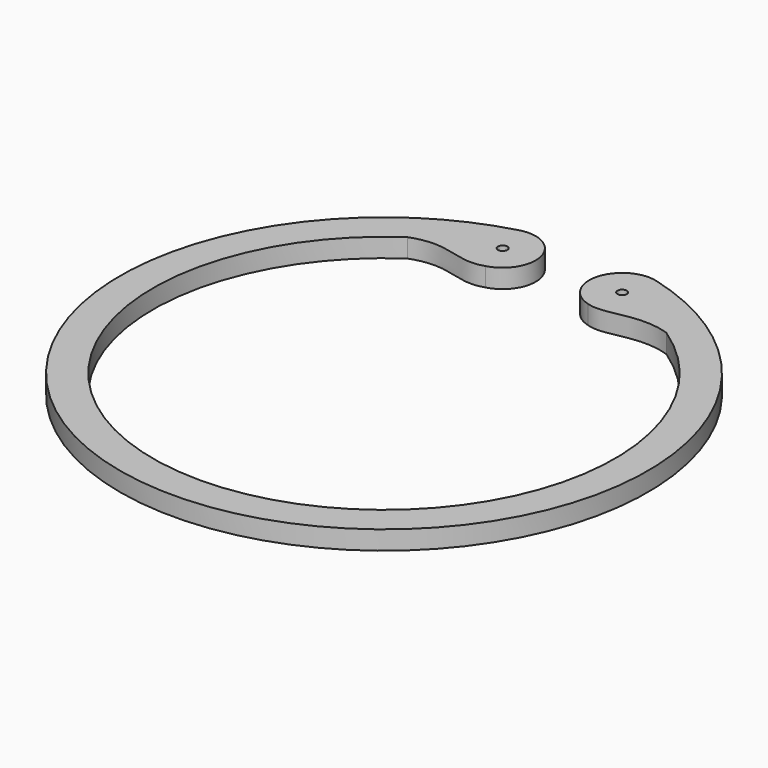
from build123d import *

# Parameters (mm, degrees)
F1_DEPTH = 1
F2_D     = 0.5
F2_DEPTH = 17
F2_TIP   = 0.1502151548


with BuildPart() as f1:
    # F0 (on Top) → F1 (new body)
    with BuildSketch(Plane.XY):
        with BuildLine():
            add(Edge.make_bspline(
                [(-6.8700691129, 10.142221176), (-8.399545307, 9.5712927005), (-10.6213726103, 7.7990288846), (-9.4482654422, 10.3310348046)],
                knots=[0.5589666429, 0.5589666429, 0.5589666429, 0.5589666429, 1, 1, 1, 1], degree=3))
            add(Edge.make_bspline(
                [(-2.7175999736, 10.142221176), (-4.1052754968, 9.659698233), (-4.9316076337, 10.8658171767), (-6.8700691129, 10.142221176)],
                knots=[0, 0, 0, 0, 0.5589666429, 0.5589666429, 0.5589666429, 0.5589666429], degree=3))
            Line((-2.7175999736, 10.142221176), (-3.6234666314, 13.522961568))
            ThreePointArc((-3.6234666314, 13.522961568), (-6.727900413, 12.2774327949), (-9.4482654422, 10.3310348046))
        make_face()
        with BuildLine():
            ThreePointArc((6.8700691129, 10.142221176), (0, -12.25), (-6.8700691129, 10.142221176))
            add(Edge.make_bspline(
                [(-6.8700691129, 10.142221176), (-8.399545307, 9.5712927005), (-10.6213726103, 7.7990288846), (-9.4482654422, 10.3310348046)],
                knots=[0.5589666429, 0.5589666429, 0.5589666429, 0.5589666429, 1, 1, 1, 1], degree=3))
            ThreePointArc((-9.4482654422, 10.3310348046), (0, -14), (9.4482654422, 10.3310348046))
            add(Edge.make_bspline(
                [(6.8700691129, 10.142221176), (8.3520722793, 9.6407168218), (10.2458875626, 8.1284232438), (9.4482654422, 10.3310348046)],
                knots=[0.5589666429, 0.5589666429, 0.5589666429, 0.5589666429, 1, 1, 1, 1], degree=3))
        make_face()
        with BuildLine():
            add(Edge.make_bspline(
                [(2.7175999736, 10.142221176), (3.7749782205, 9.7897974774), (4.9917750531, 10.7778288933), (6.8700691129, 10.142221176)],
                knots=[0, 0, 0, 0, 0.5589666429, 0.5589666429, 0.5589666429, 0.5589666429], degree=3))
            add(Edge.make_bspline(
                [(6.8700691129, 10.142221176), (8.3520722793, 9.6407168218), (10.2458875626, 8.1284232438), (9.4482654422, 10.3310348046)],
                knots=[0.5589666429, 0.5589666429, 0.5589666429, 0.5589666429, 1, 1, 1, 1], degree=3))
            ThreePointArc((9.4482654422, 10.3310348046), (6.727900413, 12.2774327949), (3.6234666314, 13.522961568))
            Line((3.6234666314, 13.522961568), (2.7175999736, 10.142221176))
        make_face()
        with BuildLine():
            Line((-3.6234666314, 13.522961568), (-2.7175999736, 10.142221176))
            ThreePointArc((-2.7175999736, 10.142221176), (-1.4801631065, 12.285524701), (-3.6234666314, 13.522961568))
        make_face()
        with BuildLine():
            ThreePointArc((3.6234666314, 13.522961568), (1.4801631065, 12.285524701), (2.7175999736, 10.142221176))
            Line((2.7175999736, 10.142221176), (3.6234666314, 13.522961568))
        make_face()
    extrude(amount=F1_DEPTH)

    # F2
    with Locations(Plane(origin=(0, 0, 0), x_dir=(1, 0, 0), z_dir=(0, 0, -1))):
        with Locations((-3.1705333025, -11.832591372), (3.1705333025, -11.832591372)):
            Hole(F2_D / 2, depth=F2_DEPTH)
            with Locations((0, 0, -(F2_DEPTH + F2_TIP / 2))):  # 118° drill point
                Cone(0, F2_D / 2, F2_TIP, mode=Mode.SUBTRACT)


solid = f1.part
